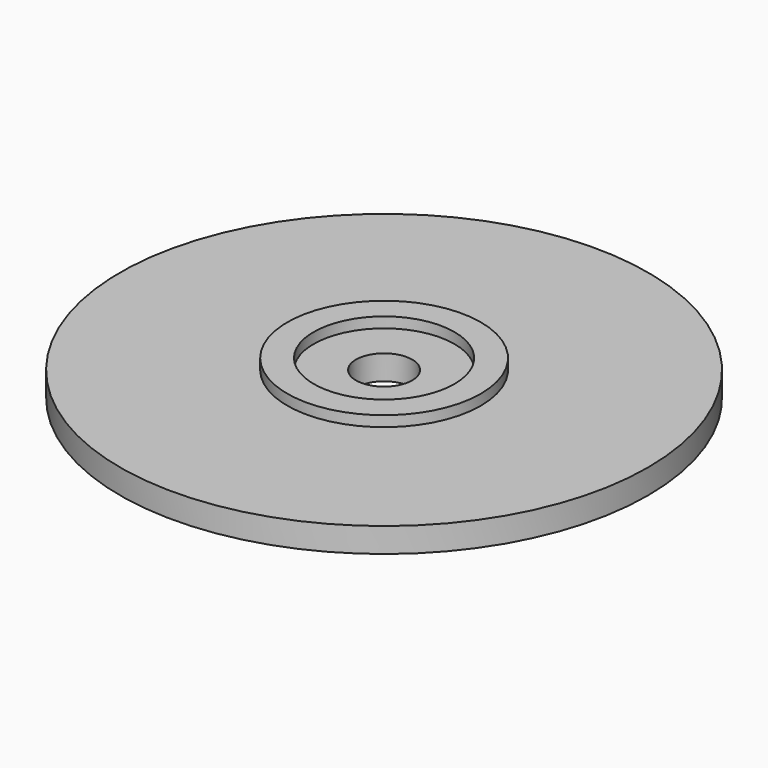
from build123d import *

# Parameters (mm, degrees)
F0_R     = 15
F0_R_2   = 1.6
F1_DEPTH = 1.4
F2_R     = 5.5
F2_R_2   = 4
F3_DEPTH = 0.6


# Not quite as in the source:
# - a feature names something its author has since deleted; it is built from what else it names


with BuildPart() as f1:
    # F0 (on Top) → F1 (new body)
    with BuildSketch(Plane.XY):
        Circle(F0_R)
        Circle(F0_R_2, mode=Mode.SUBTRACT)
    extrude(amount=F1_DEPTH)

    # F2 (on face) → F3 (join)
    with BuildSketch(Plane.XY.offset(1.4)):
        Circle(F2_R)
        Circle(F2_R_2, mode=Mode.SUBTRACT)
    extrude(amount=F3_DEPTH)


solid = f1.part
